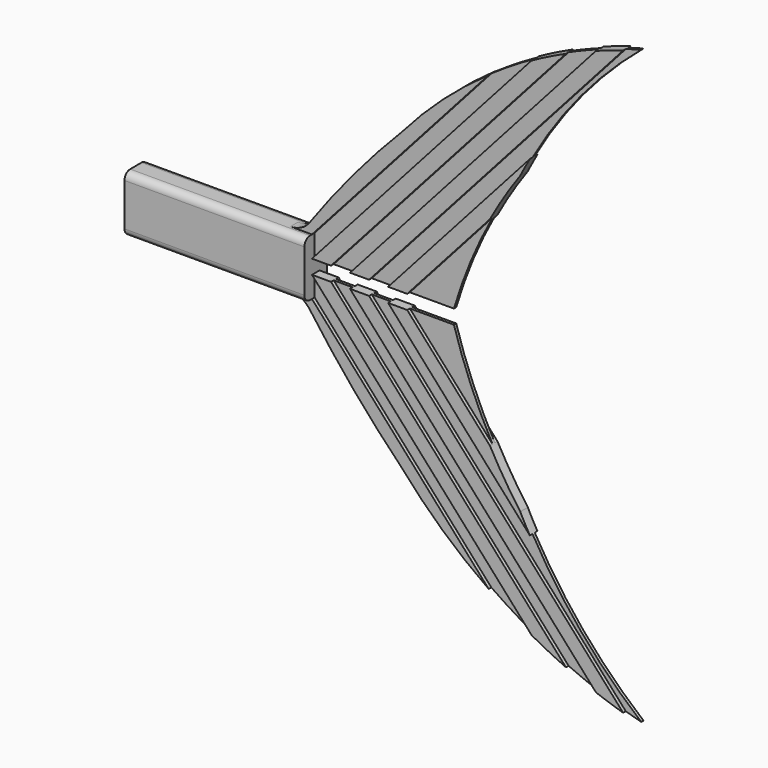
from build123d import *

# Parameters (mm, degrees)
F1_DEPTH         = 1
F3_W             = 38
F3_H             = 12
F4_DEPTH         = 3
F5_R             = 1.5
F7_DEPTH         = 0.7
F7_COPIES2_COUNT = 2
F9_DEPTH         = 12.5
F10_R            = 5


# Not quite as in the source:
# - a pattern or mirror of a feature is missing from the dataset's text; its kind, count and spacing are read off the source's solid


with BuildPart() as f1:
    # F0 (on Front) → F1 (new body, symmetric)
    with BuildSketch(Plane.XZ):
        with BuildLine():
            ThreePointArc((25, 31.25), (11.7164027855, 16.2518777716), (0, 0))
            Line((0, 0), (35, 0))
            ThreePointArc((35, 0), (41.1356304071, 16.2798974046), (50, 31.25))
            Line((50, 31.25), (25, 31.25))
        make_face()
        with BuildLine():
            ThreePointArc((75, 62.5), (47.6444357815, 50.6439027497), (25, 31.25))
            Line((25, 31.25), (50, 31.25))
            ThreePointArc((50, 31.25), (60.9207680237, 48.138385581), (75, 62.5))
        make_face()
    extrude(amount=F1_DEPTH, both=True)

    # F2: F1 across plane


with BuildPart() as f1_1:
    add(f1.part)
    add(f1.part.mirror(Plane.XY))

    # F3 (on Front) → F4 (join, symmetric)
    with BuildSketch(Plane.XZ):
        with Locations((-13, 0)):
            Rectangle(F3_W, F3_H)
    extrude(amount=F4_DEPTH, both=True)

    # F5
    f5_edges = [f1_1.edges().sort_by_distance(p)[0] for p in [
        (-13, 3, 6),
        (-13, -3, 6),
        (-13, -3, -6),
        (-13, 3, -6),
    ]]
    fillet(f5_edges, radius=F5_R)

    # F6 (on face) → F7 (cut)
    with BuildSketch(Plane.XZ.offset(1)):
        with BuildLine():
            Line((43.3365657685, 47.794180243), (6, 6))
            Line((6, 6), (6, 1.5))
            Line((6, 1.5), (6.0027095677, 1.5))
            Line((6.0027095677, 1.5), (52.4002239395, 53.436915958))
            ThreePointArc((52.4002239395, 53.436915958), (47.7930343948, 50.7365960242), (43.3365657685, 47.794180243))
        make_face()
        with BuildLine():
            ThreePointArc((65.9958136081, 59.6496176381), (62.8051828619, 58.40863879), (59.6589001751, 57.0591728532))
            Line((59.6589001751, 57.0591728532), (10.0254655864, 1.5))
            Line((10.0254655864, 1.5), (14.0482216051, 1.5))
            Line((14.0482216051, 1.5), (65.9958136081, 59.6496176381))
        make_face()
        with BuildLine():
            ThreePointArc((75, 62.5), (73.3655345805, 62.0514906305), (71.738905371, 61.5753443538))
            Line((71.738905371, 61.5753443538), (18.0709776237, 1.5))
            Line((18.0709776237, 1.5), (22.0937336424, 1.5))
            Line((22.0937336424, 1.5), (52.0251632611, 35.0049445138))
            ThreePointArc((52.0251632611, 35.0049445138), (62.2710885073, 49.7898624827), (75, 62.5))
        make_face()
        with BuildLine():
            Line((43.5901115949, 21.0597985398), (26.1164896611, 1.5))
            Line((26.1164896611, 1.5), (35.4331656898, 1.5))
            ThreePointArc((35.4331656898, 1.5), (38.9920250058, 11.4965917024), (43.5901115949, 21.0597985398))
        make_face()
    f7 = extrude(amount=-F7_DEPTH, mode=Mode.SUBTRACT)

    # F7_copies: F7 across plane
    add(f7.mirror(Plane.ZX), mode=Mode.SUBTRACT)

    # F7_copies1: F7 across plane
    add(f7.mirror(Plane(origin=(0, 0, 0), x_dir=(-1, 0, 0), z_dir=(0, 0, -1))), mode=Mode.SUBTRACT)

    # F7_copies2: F7 ×2 about axis
    f7_copies2_axis = Axis((0, 0, 0), (1, 0, 0))
    for i in range(1, F7_COPIES2_COUNT):
        add(f7.rotate(f7_copies2_axis, i * 360 / F7_COPIES2_COUNT), mode=Mode.SUBTRACT)

    # F8 (on face) → F9 (cut, symmetric)
    with BuildSketch(Plane.XZ.offset(1)):
        with BuildLine():
            Line((6.0027095677, 1.5), (6, 1.5))
            Line((6, 1.5), (6, -1.5))
            Line((6, -1.5), (6.0027095677, -1.5))
            Line((6.0027095677, -1.5), (10.0254655864, -1.5))
            Line((10.0254655864, -1.5), (14.0482216051, -1.5))
            Line((14.0482216051, -1.5), (18.0709776237, -1.5))
            Line((18.0709776237, -1.5), (22.0937336424, -1.5))
            Line((22.0937336424, -1.5), (26.1164896611, -1.5))
            Line((26.1164896611, -1.5), (35.4331656898, -1.5))
            ThreePointArc((35.4331656898, -1.5), (35.2136553779, -0.7508453855), (35, 0))
            ThreePointArc((35, 0), (35.2136553779, 0.7508453855), (35.4331656898, 1.5))
            Line((35.4331656898, 1.5), (26.1164896611, 1.5))
            Line((26.1164896611, 1.5), (22.0937336424, 1.5))
            Line((22.0937336424, 1.5), (18.0709776237, 1.5))
            Line((18.0709776237, 1.5), (14.0482216051, 1.5))
            Line((14.0482216051, 1.5), (10.0254655864, 1.5))
            Line((10.0254655864, 1.5), (6.0027095677, 1.5))
        make_face()
    extrude(amount=F9_DEPTH, both=True, mode=Mode.SUBTRACT)

    # F10
    f10_edges = [f1_1.edges().sort_by_distance(p)[0] for p in [
        (4.040045, 0, 6),
        (4.040045, 0, -6),
    ]]
    fillet(f10_edges, radius=F10_R)


solid = f1_1.part
